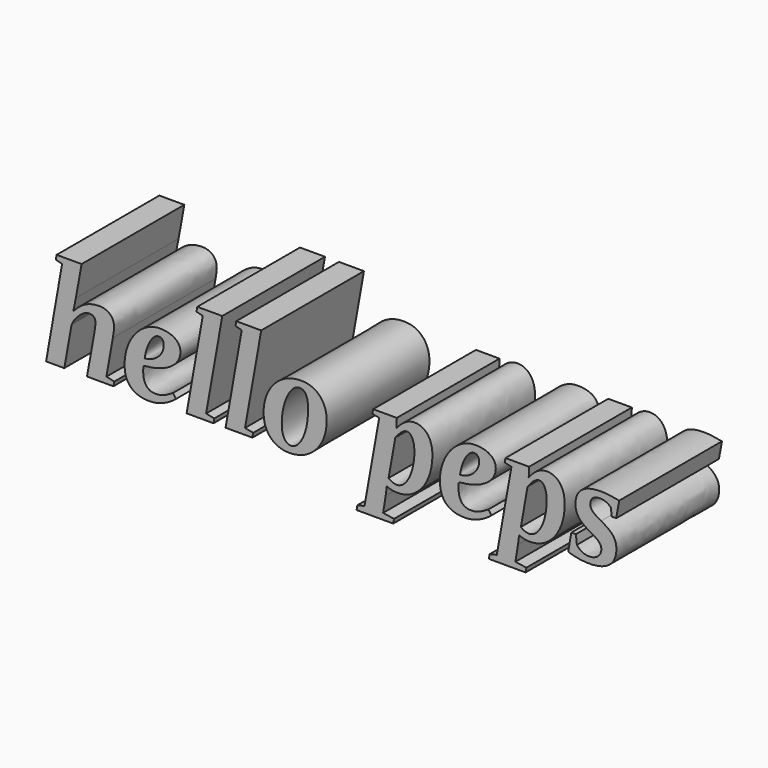
from build123d import *

# Parameters (mm, degrees)
F0_TEXT_SIZE = 27.2927909262
F1_DEPTH     = 25


# Not quite as in the source:
# - Text() gives the source's letters only with a copy of the font that has no kerning and outlines rounded to 1/6400 em; it was checked with that copy


with BuildPart() as f1:
    # F0 (on Front) → F1 (new body)
    with BuildSketch(Plane.XZ):
        with Locations((-27.6704914868, 19.0061852336)):
            Text('hello peps', F0_TEXT_SIZE, font='Tinos', font_style=FontStyle.BOLDITALIC, text_align=(TextAlign.LEFT, TextAlign.BOTTOM))
    extrude(amount=F1_DEPTH)


solid = f1.part
